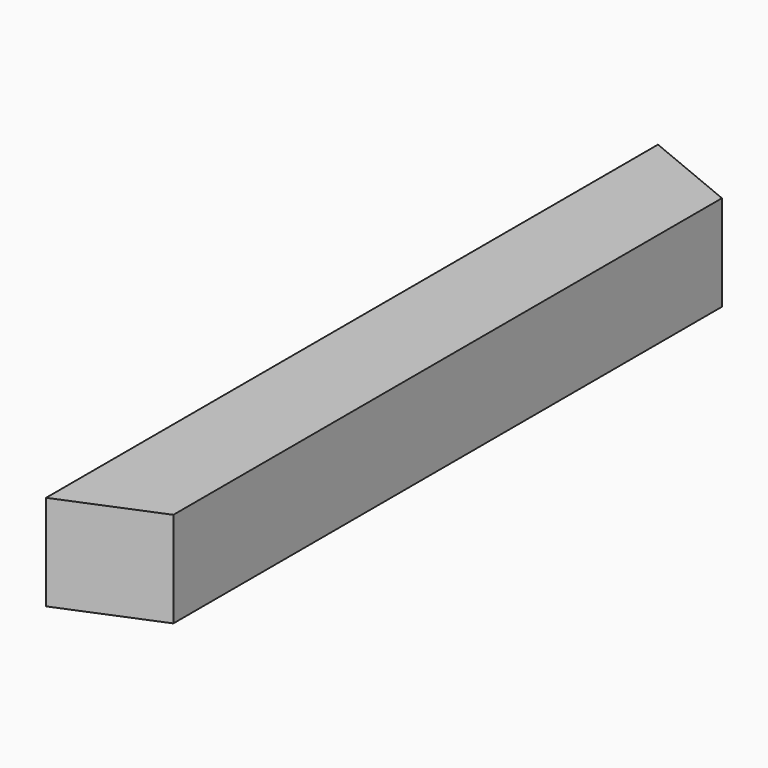
from build123d import *

# Parameters (mm, degrees)
F0_W       = 25.4
F0_H       = 25.4
F1_DEPTH   = 101.6
F2_SIZE2   = 10.521014
F2_SIZE    = 25.39999
F2_2_SIZE2 = 10.521014
F2_2_SIZE  = 25.39999


# Not quite as in the source:
# - a fillet or chamfer is up to 0.001 mm smaller than in the source, because OpenCascade refuses the exact size


with BuildPart() as f1:
    # F0 (on Front) → F1 (new body, symmetric)
    with BuildSketch(Plane.XZ):
        Rectangle(F0_W, F0_H)
    extrude(amount=F1_DEPTH, both=True)

    # F2 (size 25.4 and 10.5210244843 in the source; OpenCascade refuses exactly that, so slightly less here)
    f2_edges = [f1.edges().sort_by_distance(p)[0] for p in [
        (12.7, -101.6, 0),
    ]]
    f2_side = f1.faces().sort_by_distance((0, -101.6, 0))[0]
    chamfer(f2_edges, length=F2_SIZE, length2=F2_SIZE2, reference=f2_side)

    # F2#2 (size 25.4 and 10.5210244843 in the source; OpenCascade refuses exactly that, so slightly less here)
    f2_2_edges = [f1.edges().sort_by_distance(p)[0] for p in [
        (12.7, 101.6, 0),
    ]]
    f2_2_side = f1.faces().sort_by_distance((0, 101.6, 0))[0]
    chamfer(f2_2_edges, length=F2_2_SIZE, length2=F2_2_SIZE2, reference=f2_2_side)


solid = f1.part
